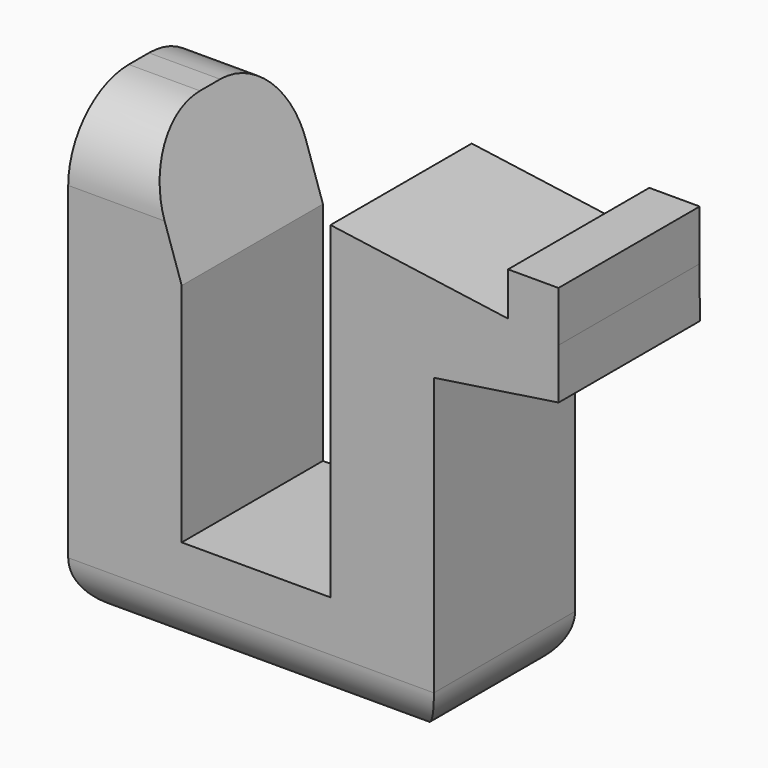
from build123d import *

# Parameters (mm, degrees)
F1_DEPTH = 3.5
F2_R     = 3
F3_R     = 2


with BuildPart() as f1:
    # F0 (on Front) → F1 (new body, symmetric)
    with BuildSketch(Plane.XZ):
        Polygon((-6.367480836, -8.9669886286), (-12.267480836, -8.9669886286), (-12.267480836, 0), (-13.942480836, 5.0330113714), (-15.617480836, 5.0330113714), (-16.767480836, 5.0330113714), (-16.767480836, 0.0330113714), (-16.767480836, -12.9669886286), (-2.267480836, -12.9669886286), (-2.267480836, -3.9669886286), (-2.267480836, 0.0330113714), (2.6771662389, 0.7749448625), (2.6740676862, 2.7749424623), (2.6740676862, 4.7749424623), (0.6740676862, 4.7749424623), (0.6740676862, 3.0532286222), (-6.367480836, 4.0330113714), (-6.367480836, 0.0330113714), align=None)
    extrude(amount=F1_DEPTH, both=True)

    # F2
    f2_edges = [f1.edges().sort_by_distance(p)[0] for p in [
        (-15.354981, 3.5, 5.033011),
        (-15.354981, -3.5, 5.033011),
    ]]
    fillet(f2_edges, radius=F2_R)

    # F3
    f3_edges = [f1.edges().sort_by_distance(p)[0] for p in [
        (-16.767481, 0, -12.966989),
        (-9.517481, 3.5, -12.966989),
        (-2.267481, 0, -12.966989),
        (-9.517481, -3.5, -12.966989),
    ]]
    fillet(f3_edges, radius=F3_R)


solid = f1.part
